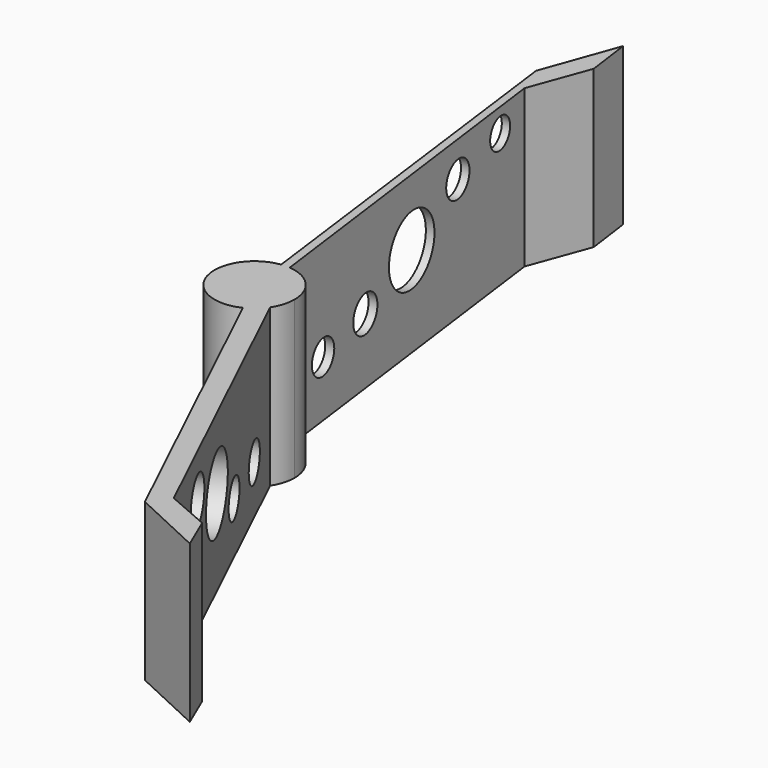
from build123d import *

# Parameters (mm, degrees)
F1_DEPTH = 500
F2_R     = 48.0212425181
F2_R_2   = 56.0010929185
F2_R_3   = 109.5030020502
F2_R_4   = 58.0607354524
F2_R_5   = 53.7611851769
F3_DEPTH = 50
F5_DEPTH = 500
F6_R     = 60.7396670844
F6_R_2   = 74.2371640954
F6_R_3   = 52.0726222856
F6_R_4   = 59.6000564376
F6_R_5   = 119.2001237969
F7_DEPTH = 100


# Not quite as in the source:
# - a feature names something its author has since deleted; it is built from what else it names


with BuildPart() as f1:
    # F0 (on Top) → F1 (new body)
    with BuildSketch(Plane.XY):
        with BuildLine():
            ThreePointArc((-16.3297786736, 125.9457753498), (-2.847496792, 126.9680737903), (10.6670605483, 126.5512300187))
            Line((10.6670605483, 126.5512300187), (-137.3067498207, 1246.1612224579))
            Line((-137.3067498207, 1246.1612224579), (-68.1192024335, 1435.3577301921))
            Line((-68.1192024335, 1435.3577301921), (-87.3996093869, 1576.3362646103))
            Line((-87.3996093869, 1576.3362646103), (-173.4057664871, 1337.4170064926))
            Line((-173.4057664871, 1337.4170064926), (-16.3297786736, 125.9457753498))
        make_face()
        with BuildLine():
            ThreePointArc((-16.3297786736, 125.9457753498), (-83.8305377188, -95.4014724508), (127, 0))
            ThreePointArc((127, 0), (93.4979055638, 85.9484825647), (10.6670605483, 126.5512300187))
            ThreePointArc((10.6670605483, 126.5512300187), (-2.847496792, 126.9680737903), (-16.3297786736, 125.9457753498))
        make_face()
    extrude(amount=F1_DEPTH)

    # F2 (on face) → F3 (cut)
    with BuildSketch(Plane(origin=(0, 0, 0), x_dir=(0.1285809344, -0.9916990185, 0), z_dir=(-0.9916990185, -0.1285809344, 0))):
        with Locations((-1136.4312171936, 425.6200194359)):
            Circle(F2_R)
        with Locations((-933.0058097839, 387.370377779)):
            Circle(F2_R_2)
        with Locations((-711.0854387283, 287.7508103848)):
            Circle(F2_R_3)
        with Locations((-487.9950881004, 208.4301263094)):
            Circle(F2_R_4)
        with Locations((-284.7935259342, 177.8837442398)):
            Circle(F2_R_5)
    extrude(amount=-F3_DEPTH, mode=Mode.SUBTRACT)

    # F4 (on face) → F5 (join)
    with BuildSketch(Plane(origin=(0, 0, 0), x_dir=(1, 0, 0), z_dir=(0, 0, -1))):
        with BuildLine():
            Line((517.1427625415, 1082.8496493747), (54.8823102258, 114.918538341))
            ThreePointArc((54.8823102258, 114.918538341), (83.4911676886, 96.1642519242), (106.0759476154, 70.4714961361))
            Line((106.0759476154, 70.4714961361), (560.7657432556, 1022.5503444672))
            Line((560.7657432556, 1022.5503444672), (699.5562911034, 1082.8496493747))
            Line((699.5562911034, 1082.8496493747), (744.8581457138, 1188.7502670288))
            Line((744.8581457138, 1188.7502670288), (517.1427625415, 1082.8496493747))
        make_face()
        with BuildLine():
            ThreePointArc((106.0759476154, 70.4714961361), (83.4911676886, 96.1642519242), (54.8823102258, 114.918538341))
            ThreePointArc((54.8823102258, 114.918538341), (-107.7210952255, -67.9301411273), (127.3512403951, 0))
            ThreePointArc((127.3512403951, 0), (121.9164507666, 36.8064866923), (106.0759476154, 70.4714961361))
        make_face()
    extrude(amount=-F5_DEPTH)

    # F6 (on face) → F7 (cut)
    with BuildSketch(Plane(origin=(0, 0, 0), x_dir=(0.4309523021, -0.9023747078, 0), z_dir=(-0.9023747078, -0.4309523021, 0))):
        with Locations((282.9372286797, 154.2636454105)):
            Circle(F6_R)
        with Locations((903.6465287209, 359.3041300774)):
            Circle(F6_R_2)
        with Locations((1114.4098043442, 373.2200860977)):
            Circle(F6_R_3)
        with Locations((504.1354894638, 163.9334559441)):
            Circle(F6_R_4)
        with Locations((692.0155882835, 273.2473611832)):
            Circle(F6_R_5)
    extrude(amount=-F7_DEPTH, mode=Mode.SUBTRACT)


solid = f1.part
